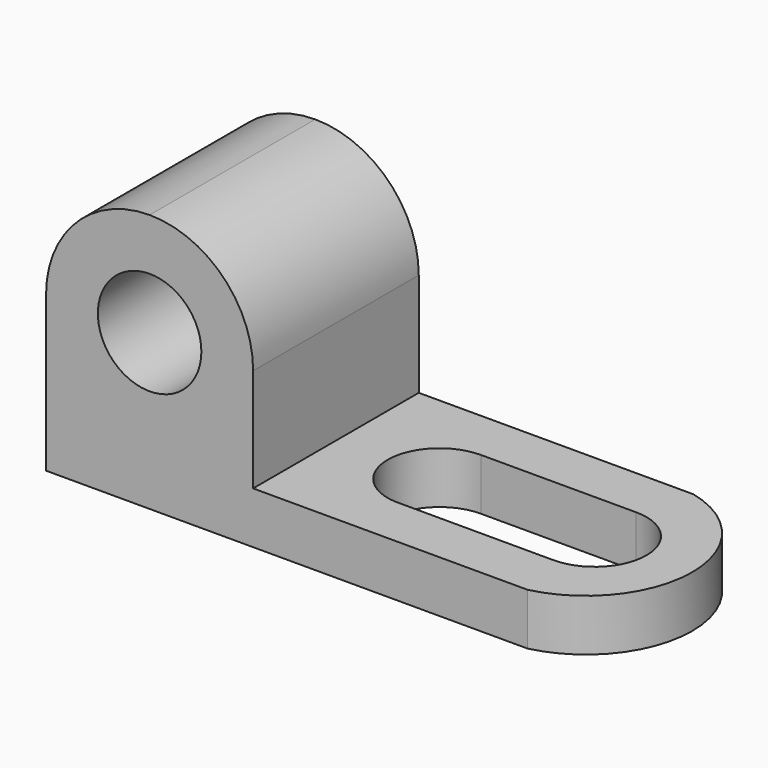
from build123d import *

# Parameters (mm, degrees)
F0_W      = 69.85
F0_H      = 31.75
F1_DEPTH  = 25.4
F2_W      = 44.45
F2_H      = 25.4
F3_DEPTH  = 25.4
F4_R      = 12.69999
F5_R      = 6.35
F7_DEPTH  = 25.4
F8_DEPTH  = 25.4
F10_DEPTH = 25.4
F11_R     = 6.35
F12_DEPTH = 25.4
F14_DEPTH = 25.4


# Not quite as in the source:
# - a fillet or chamfer is up to 0.001 mm smaller than in the source, because OpenCascade refuses the exact size
# - ends of sketch curves that miss each other by under 0.0002 mm in the source are joined


with BuildPart() as f1:
    # F0 (on Front) → F1 (new body)
    with BuildSketch(Plane.XZ):
        with Locations((34.925, 15.875)):
            Rectangle(F0_W, F0_H)
    extrude(amount=F1_DEPTH)

    # F2 (on face) → F3 (cut)
    with BuildSketch(Plane.XZ.offset(25.4)):
        with Locations((47.625, 19.05)):
            Rectangle(F2_W, F2_H)
    extrude(amount=-F3_DEPTH, mode=Mode.SUBTRACT)

    # F4 (radius 12.7 in the source; OpenCascade refuses exactly that, so slightly less here)
    f4_edges = [f1.edges().sort_by_distance(p)[0] for p in [
        (25.4, -12.7, 31.75),
        (0, -12.7, 31.75),
    ]]
    fillet(f4_edges, radius=F4_R)

    # F5 (on face) → F7 (cut)
    with BuildSketch(Plane.XY.offset(6.35)):
        with Locations((38.1, -12.7)):
            Circle(F5_R)
    extrude(amount=-F7_DEPTH, mode=Mode.SUBTRACT)

    # F6 (on face) → F8 (cut)
    with BuildSketch(Plane.XY.offset(6.35)):
        with BuildLine():
            ThreePointArc((57.15, -19.05), (61.6401280605, -17.1901280605), (63.5, -12.7))
            ThreePointArc((63.5, -12.7), (61.6401280605, -8.2098719395), (57.15, -6.35))
            Line((57.15, -6.35), (38.1, -6.35))
            ThreePointArc((38.1, -6.35), (42.5901280605, -8.2098719395), (44.45, -12.7))
            ThreePointArc((44.45, -12.7), (42.7293038012, -17.046498167), (38.4997491919, -19.0374048777))
            Line((38.4997491919, -19.0374048777), (57.15, -19.05))
        make_face()
    extrude(amount=-F8_DEPTH, mode=Mode.SUBTRACT)

    # F9 (on face) → F10 (cut)
    with BuildSketch(Plane.XY.offset(6.35)):
        with BuildLine():
            ThreePointArc((63.8472363353, 0), (69.4711968718, -12.5871403191), (64.3824189901, -25.4))
            Line((64.3824189901, -25.4), (69.85, -25.4))
            Line((69.85, -25.4), (69.85, 0))
            Line((69.85, 0), (63.8472363353, 0))
        make_face()
    extrude(amount=-F10_DEPTH, mode=Mode.SUBTRACT)

    # F11 (on face) → F12 (cut)
    with BuildSketch(Plane.XZ.offset(25.4)):
        with Locations((12.7, 19.05)):
            Circle(F11_R)
    extrude(amount=-F12_DEPTH, mode=Mode.SUBTRACT)

    # F13 (on face) → F14 (cut)
    with BuildSketch(Plane.XY.offset(6.35)):
        with BuildLine():
            ThreePointArc((59.0771511197, 0), (69.1111732298, -12.7), (59.0771511197, -25.4))
            Line((59.0771511197, -25.4), (64.3824189901, -25.4))
            ThreePointArc((64.3824189901, -25.4), (69.4711968718, -12.5871403191), (63.8472363353, 0))
            Line((63.8472363353, 0), (59.0771511197, 0))
        make_face()
    extrude(amount=-F14_DEPTH, mode=Mode.SUBTRACT)


solid = f1.part
